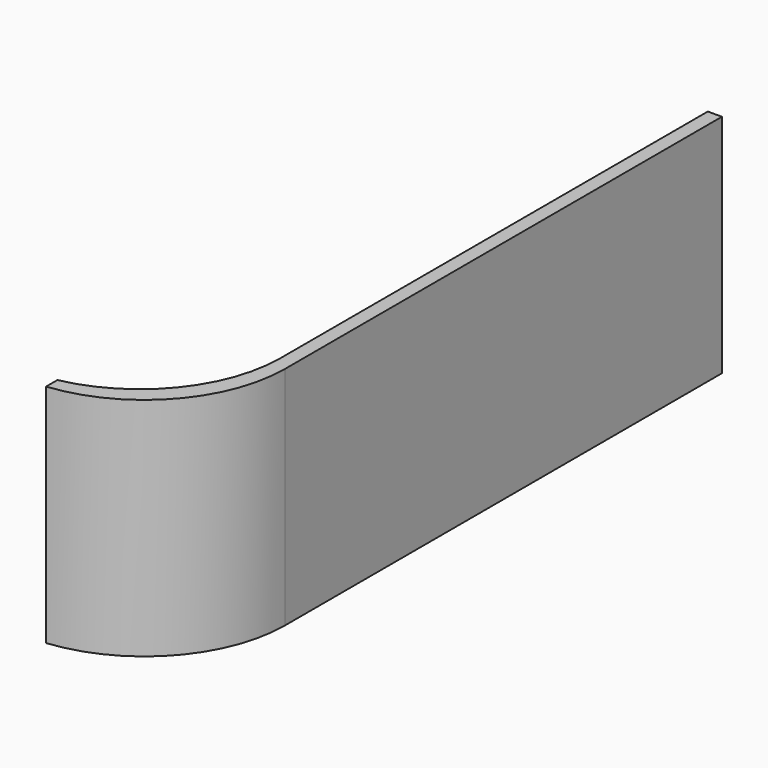
from build123d import *

# Parameters (mm, degrees)
F0_W        = 5
F0_H        = 5
F0_W_2      = 40
F0_H_2      = 238
F1_DEPTH    = 80
F2_T4_DEPTH = 80
F2_T7_DEPTH = 328.751226723


# Not quite as in the source:
# - a fillet or chamfer that OpenCascade refuses, or shapes differently, is made with other operations: its cross-section is extruded or revolved along the edge and cut away or added


with BuildPart() as f1:
    # F0 (on Top) → F1 (new body)
    with BuildSketch(Plane.XY):
        with Locations((0, -119)):
            Rectangle(F0_W, F0_H)
        with Locations((-22.5, -119)):
            Rectangle(F0_W_2, F0_H)
        with Locations((0, 2.5)):
            Rectangle(F0_W, F0_H_2)
    extrude(amount=F1_DEPTH)

    # F2: fillet of radius 50 on 2 edges, made by hand


with BuildPart() as f2_tool2:
    # F2_s3 → F2_t4 (new body)
    with BuildSketch(Plane.XY):
        with BuildLine():
            ThreePointArc((-2.4996, -67.5094166718), (-13.7698250279, -99.1327516284), (-42.4999199938, -116.5003919171))
            Line((-42.4999199938, -116.5003919171), (-41.4998154247, -121.3994894416))
            ThreePointArc((-41.4998154247, -121.3994894416), (-22.4999599969, -121.5001365685), (-2.5, -121.5001365685))
            Line((-2.5, -121.5001365685), (2.5001365685, -116.5))
            ThreePointArc((2.5001365685, -116.5), (2.5001365685, -92.0047083359), (2.5005365685, -67.5094166718))
            Line((2.5005365685, -67.5094166718), (-2.4996, -67.5094166718))
        make_face()
    extrude(amount=F2_T4_DEPTH)

    split(bisect_by=Plane.YZ.offset(2.5), keep=Keep.BOTTOM)

    split(bisect_by=Plane.XZ.offset(121.5), keep=Keep.BOTTOM)


with BuildPart() as f1_1:
    add(f1.part)

    # F2_t1: union F2_tool2
    add(f2_tool2.part)

    # F2_s8 → F2_t7 (cut)
    with BuildSketch(Plane.XY.offset(-124.3756133615)):
        with BuildLine():
            ThreePointArc((2.5004, -71.749754657), (-10.4186674501, -105.2913665442), (-42.499959993, -121.5003979943))
            Line((-42.499959993, -121.5003979943), (-41.9998594238, -126.475462328))
            ThreePointArc((-41.9998594238, -126.475462328), (-19.9999799965, -126.5001365685), (2.5, -126.5001365685))
            Line((2.5, -126.5001365685), (7.5001365685, -121.5))
            ThreePointArc((7.5001365685, -121.5), (7.5001365685, -96.6248773285), (7.5005365685, -71.749754657))
            Line((7.5005365685, -71.749754657), (2.5004, -71.749754657))
        make_face()
    extrude(amount=F2_T7_DEPTH, mode=Mode.SUBTRACT)


solid = f1_1.part
